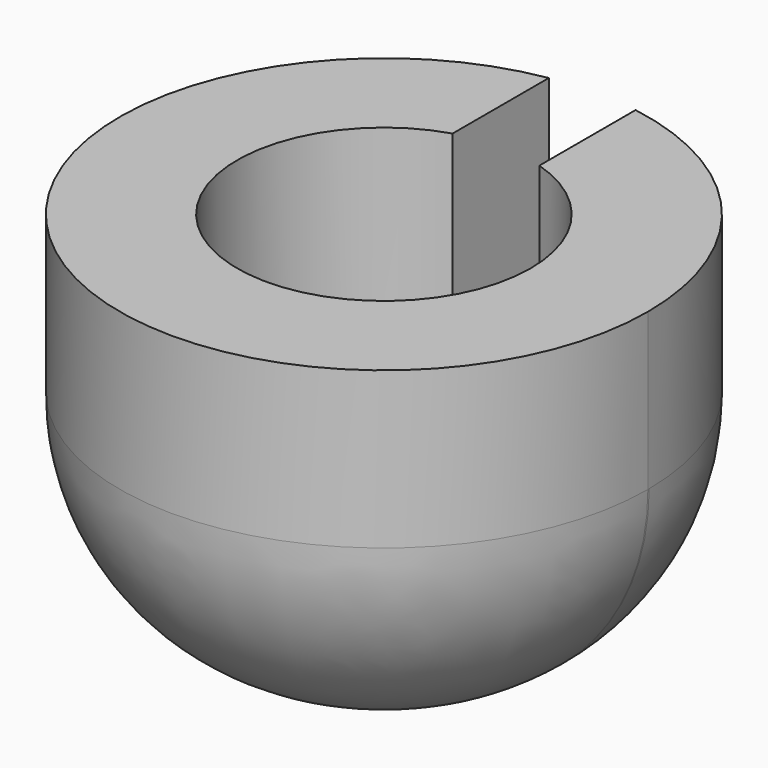
from build123d import *

# Parameters (mm, degrees)
F1_DEPTH    = 10
F2_DEPTH    = 5
F3_T2_ANGLE = 359.64
F3_T4_ANGLE = 207.9069363925


# Not quite as in the source:
# - a fillet or chamfer that OpenCascade refuses, or shapes differently, is made with other operations: its cross-section is extruded or revolved along the edge and cut away or added


with BuildPart() as f1:
    # F0 (on Top) → F1 (new body)
    with BuildSketch(Plane.XY):
        with BuildLine():
            ThreePointArc((1.1091883061, 3.5822062059), (3.0184396754, 2.2252015473), (3.75, 0))
            ThreePointArc((3.75, 0), (-2.2252015473, -3.0184396754), (-1.1091883061, 3.5822062059))
            Line((-1.1091883061, 3.5822062059), (-1.1091883061, 6.6582431092))
            ThreePointArc((-1.1091883061, 6.6582431092), (-4.3632258097, -5.1502194646), (6.75, 0))
            ThreePointArc((6.75, 0), (5.1502194646, 4.3632258097), (1.1091883061, 6.6582431092))
            Line((1.1091883061, 6.6582431092), (1.1091883061, 3.5822062059))
        make_face()
    extrude(amount=F1_DEPTH)

    # F0 (on Top) → F2 (join)
    with BuildSketch(Plane.XY):
        with BuildLine():
            ThreePointArc((-1.1091883061, 3.5822062059), (-2.2252015473, -3.0184396754), (3.75, 0))
            ThreePointArc((3.75, 0), (3.0184396754, 2.2252015473), (1.1091883061, 3.5822062059))
            Line((1.1091883061, 3.5822062059), (1.1091883061, 0.75))
            Line((1.1091883061, 0.75), (-1.1091883061, 0.75))
            Line((-1.1091883061, 0.75), (-1.1091883061, 3.5822062059))
        make_face()
        with BuildLine():
            Line((1.1091883061, 0.75), (1.1091883061, 3.5822062059))
            ThreePointArc((1.1091883061, 3.5822062059), (0, 3.75), (-1.1091883061, 3.5822062059))
            Line((-1.1091883061, 3.5822062059), (-1.1091883061, 0.75))
            Line((-1.1091883061, 0.75), (1.1091883061, 0.75))
        make_face()
    extrude(amount=F2_DEPTH)

    # F3: fillet of radius 6 on 1 edges, made by hand

    # F3_s1 → F3_t2 (revolve, cut)
    with BuildSketch(Plane(origin=(0, 0, 0), x_dir=(0, 0, 1), z_dir=(0.006283144, -0.9999802609, 0))):
        with BuildLine():
            ThreePointArc((6, -6.75), (1.7573593129, -4.9926406871), (0, -0.75))
            Line((0, -0.75), (0, -6.75))
            Line((0, -6.75), (6, -6.75))
        make_face()
    revolve(axis=Axis((0, 0, 0), (0, 0, 1)), revolution_arc=F3_T2_ANGLE, mode=Mode.SUBTRACT)

    # F3_s3 → F3_t4 (revolve, cut)
    with BuildSketch(Plane.XZ):
        with BuildLine():
            ThreePointArc((0.75, 0), (4.9926406871, 1.7573593129), (6.75, 6))
            Line((6.75, 6), (6.75, 0))
            Line((6.75, 0), (0.75, 0))
        make_face()
    revolve(axis=Axis((0, 0, 0), (0, 0, 1)), revolution_arc=F3_T4_ANGLE, mode=Mode.SUBTRACT)


solid = f1.part
